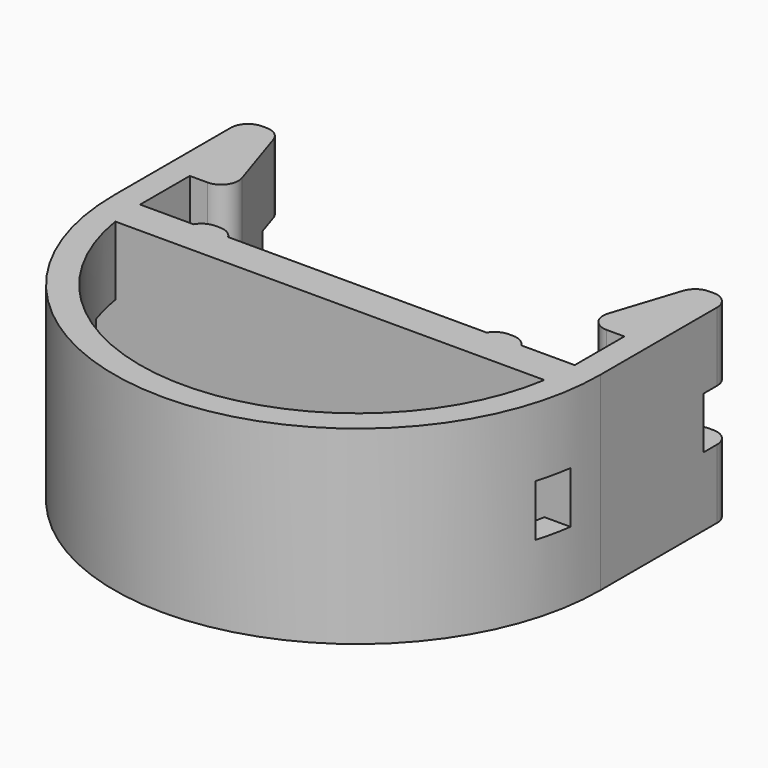
from build123d import *

# Parameters (mm, degrees)
F0_W        = 2
F0_H        = 0.5
F1_DEPTH    = 11
F2_T1_DEPTH = 17.8819096024
F2_T3_DEPTH = 16
F2_T5_DEPTH = 14.63271264
F2_T7_DEPTH = 15.3301270189
F3_W        = 2
F3_H        = 3
F4_DEPTH    = 15


# Not quite as in the source:
# - a fillet or chamfer that OpenCascade refuses, or shapes differently, is made with other operations: its cross-section is extruded or revolved along the edge and cut away or added


with BuildPart() as f1:
    # F0 (on Top) → F1 (new body)
    with BuildSketch(Plane.XY):
        with BuildLine():
            Line((-14.1, 9.4475987206), (-14.1, 0))
            ThreePointArc((-14.1, 0), (0, -14.1), (14.1, 0))
            Line((14.1, 0), (14.1, 9.4475987206))
            Line((14.1, 9.4475987206), (12.1, 9.4475987206))
            Line((12.1, 9.4475987206), (10.2, 3.6))
            Line((10.2, 3.6), (12.6, 3.6))
            Line((12.6, 3.6), (12.6, 0))
            Line((12.6, 0), (9.5, 0))
            Line((9.5, 0), (7.5, 0))
            Line((7.5, 0), (0, 0))
            Line((0, 0), (-7.5, 0))
            Line((-7.5, 0), (-9.5, 0))
            Line((-9.5, 0), (-12.6, 0))
            Line((-12.6, 0), (-12.6, 3.6))
            Line((-12.6, 3.6), (-10.2, 3.6))
            Line((-10.2, 3.6), (-12.1, 9.4475987206))
            Line((-12.1, 9.4475987206), (-14.1, 9.4475987206))
        make_face()
        with BuildLine():
            ThreePointArc((12.4402572321, -2), (0, -12.6), (-12.4402572321, -2))
            Line((-12.4402572321, -2), (12.4402572321, -2))
        make_face(mode=Mode.SUBTRACT)
        with Locations((-8.5, 0.25)):
            Rectangle(F0_W, F0_H)
        with Locations((8.5, 0.25)):
            Rectangle(F0_W, F0_H)
    extrude(amount=F1_DEPTH)

    # F2: fillet of radius 1 on 10 edges, made by hand

    # F2_s2 → F2_t1 (cut)
    with BuildSketch(Plane.XY.offset(-3.4409548012)):
        with BuildLine():
            ThreePointArc((-11.5763819205, 3.6), (-10.7673649261, 4.0122147477), (-10.6253254042, 4.9090169944))
            Line((-10.6253254042, 4.9090169944), (-10.2, 3.6))
            Line((-10.2, 3.6), (-11.5763819205, 3.6))
        make_face()
        with BuildLine():
            ThreePointArc((10.6253254042, 4.9090169944), (10.7673649261, 4.0122147477), (11.5763819205, 3.6))
            Line((11.5763819205, 3.6), (10.2, 3.6))
            Line((10.2, 3.6), (10.6253254042, 4.9090169944))
        make_face()
    extrude(amount=F2_T1_DEPTH, mode=Mode.SUBTRACT)

    # F2_s4 → F2_t3 (cut)
    with BuildSketch(Plane.XY.offset(-2.5)):
        with BuildLine():
            ThreePointArc((-13.1, 9.4475987206), (-13.8071067812, 9.1547055018), (-14.1, 8.4475987206))
            Line((-14.1, 8.4475987206), (-14.1, 9.4475987206))
            Line((-14.1, 9.4475987206), (-13.1, 9.4475987206))
        make_face()
        with BuildLine():
            ThreePointArc((14.1, 8.4475987206), (13.8071067812, 9.1547055018), (13.1, 9.4475987206))
            Line((13.1, 9.4475987206), (14.1, 9.4475987206))
            Line((14.1, 9.4475987206), (14.1, 8.4475987206))
        make_face()
    extrude(amount=F2_T3_DEPTH, mode=Mode.SUBTRACT)

    # F2_s6 → F2_t5 (cut)
    with BuildSketch(Plane.XY.offset(-1.81635632)):
        with BuildLine():
            ThreePointArc((-11.8754860117, 8.756615715), (-12.2387572757, 9.256615715), (-12.826542528, 9.4475987206))
            Line((-12.826542528, 9.4475987206), (-12.1, 9.4475987206))
            Line((-12.1, 9.4475987206), (-11.8754860117, 8.756615715))
        make_face()
        with BuildLine():
            ThreePointArc((11.8754860117, 8.756615715), (12.2387572757, 9.256615715), (12.826542528, 9.4475987206))
            Line((12.826542528, 9.4475987206), (12.1, 9.4475987206))
            Line((12.1, 9.4475987206), (11.8754860117, 8.756615715))
        make_face()
    extrude(amount=F2_T5_DEPTH, mode=Mode.SUBTRACT)

    # F2_s8 → F2_t7 (cut)
    with BuildSketch(Plane.XY.offset(-2.1650635095)):
        with BuildLine():
            ThreePointArc((-8.6339745962, 0.5), (-9.1339745962, 0.3660254038), (-9.5, 0))
            Line((-9.5, 0), (-9.5, 0.5))
            Line((-9.5, 0.5), (-8.6339745962, 0.5))
        make_face()
        with BuildLine():
            ThreePointArc((-7.5, 0), (-7.8660254038, 0.3660254038), (-8.3660254038, 0.5))
            Line((-8.3660254038, 0.5), (-7.5, 0.5))
            Line((-7.5, 0.5), (-7.5, 0))
        make_face()
        with BuildLine():
            ThreePointArc((8.3660254038, 0.5), (7.8660254038, 0.3660254038), (7.5, 0))
            Line((7.5, 0), (7.5, 0.5))
            Line((7.5, 0.5), (8.3660254038, 0.5))
        make_face()
        with BuildLine():
            ThreePointArc((9.5, 0), (9.1339745962, 0.3660254038), (8.6339745962, 0.5))
            Line((8.6339745962, 0.5), (9.5, 0.5))
            Line((9.5, 0.5), (9.5, 0))
        make_face()
    extrude(amount=F2_T7_DEPTH, mode=Mode.SUBTRACT)

    # F3 (on Right) → F4 (cut, symmetric)
    with BuildSketch(Plane.YZ):
        with Locations((-3, 5.5)):
            Rectangle(F3_W, F3_H)
        with Locations((8.4475987206, 5.5)):
            Rectangle(F3_W, F3_H)
    extrude(amount=F4_DEPTH, both=True, mode=Mode.SUBTRACT)


solid = f1.part
